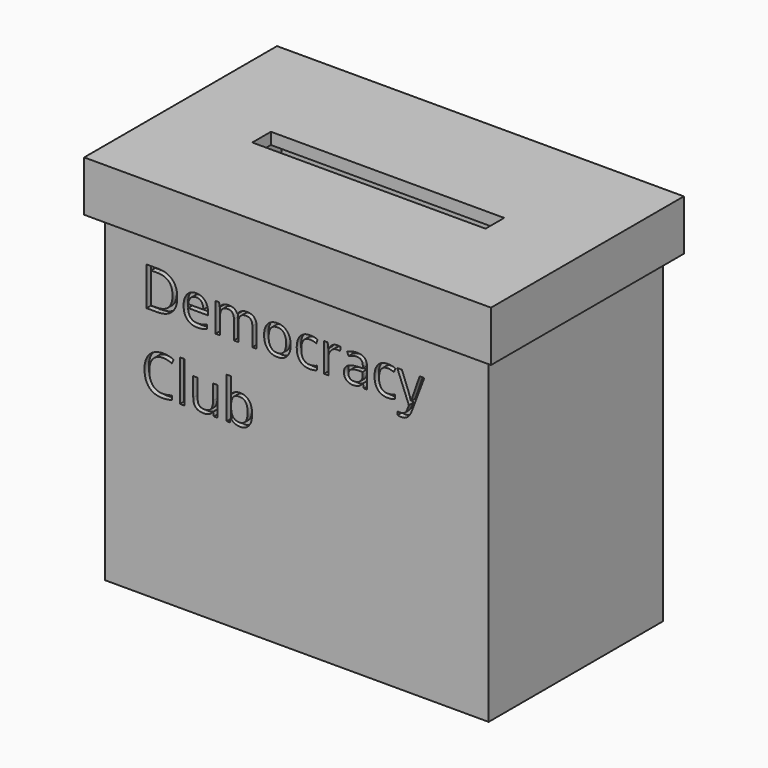
from build123d import *

# Parameters (mm, degrees)
F1_DEPTH     = 40
F2_T         = 1.5
F3_TEXT_SIZE = 6.9444444444
F4_DEPTH     = 0.7
F5_W         = 49.3177990913
F5_H         = 28
F6_DEPTH     = 5
F7_T         = 1.5
F8_DEPTH     = 74.24345


# Not quite as in the source:
# - Text() gives the source's letters only with a copy of the font that has no kerning and outlines rounded to 1/6400 em; it was checked with that copy


with BuildPart() as f1:
    # F0 (on Top) → F1 (new body)
    with BuildSketch(Plane.XY):
        Polygon((-16.0410279781, -8.8653270361), (-39.1999275237, -8.8653270361), (-39.1999275237, -33.8653270361), (7.1178715676, -33.8653270361), (7.1178715676, -8.8653270361), align=None)
        Polygon((-31.0410279781, -20.7940959632), (-16.0410279781, -20.7940959632), (-1.0410279781, -20.7940959632), (-1.0410279781, -23.7940959632), (-31.0410279781, -23.7940959632), align=None, mode=Mode.SUBTRACT)
        Polygon((-1.0410279781, -20.7940959632), (-16.0410279781, -20.7940959632), (-31.0410279781, -20.7940959632), (-31.0410279781, -23.7940959632), (-1.0410279781, -23.7940959632), align=None)
    extrude(amount=F1_DEPTH)

    # F2
    f2_openings = [f1.faces().sort_by_distance(p)[0] for p in [
        (-16.041028, -21.365327, 40),
    ]]
    offset(amount=F2_T, openings=f2_openings, kind=Kind.INTERSECTION)

    # F3 (on face) → F4 (cut)
    with BuildSketch(Plane.XZ.offset(35.3653270361)):
        with Locations((-36.0694295024, 31.0335577338)):
            Text('Democracy', F3_TEXT_SIZE, font='Open Sans', text_align=(TextAlign.LEFT, TextAlign.BOTTOM))
        with Locations((-36.0694295024, 21.5891132894)):
            Text('Club', F3_TEXT_SIZE, font='Open Sans', text_align=(TextAlign.LEFT, TextAlign.BOTTOM))
    extrude(amount=-F4_DEPTH, mode=Mode.SUBTRACT)


with BuildPart() as f6:
    # F5 (on face) → F6 (new body)
    with BuildSketch(Plane.XY.offset(40)):
        with Locations((-16.0410279781, -21.3653270361)):
            Rectangle(F5_W, F5_H)
    extrude(amount=F6_DEPTH)

    # F7
    f7_openings = [f6.faces().sort_by_distance(p)[0] for p in [
        (-16.041028, -21.365327, 40),
    ]]
    offset(amount=F7_T, openings=f7_openings, kind=Kind.INTERSECTION)

    # F0 (on Top) → F8 (cut)
    with BuildSketch(Plane.XY):
        Polygon((-1.0410279781, -20.7940959632), (-16.0410279781, -20.7940959632), (-31.0410279781, -20.7940959632), (-31.0410279781, -23.7940959632), (-1.0410279781, -23.7940959632), align=None)
    extrude(amount=F8_DEPTH, mode=Mode.SUBTRACT)


solid = Compound([f1.part, f6.part])
